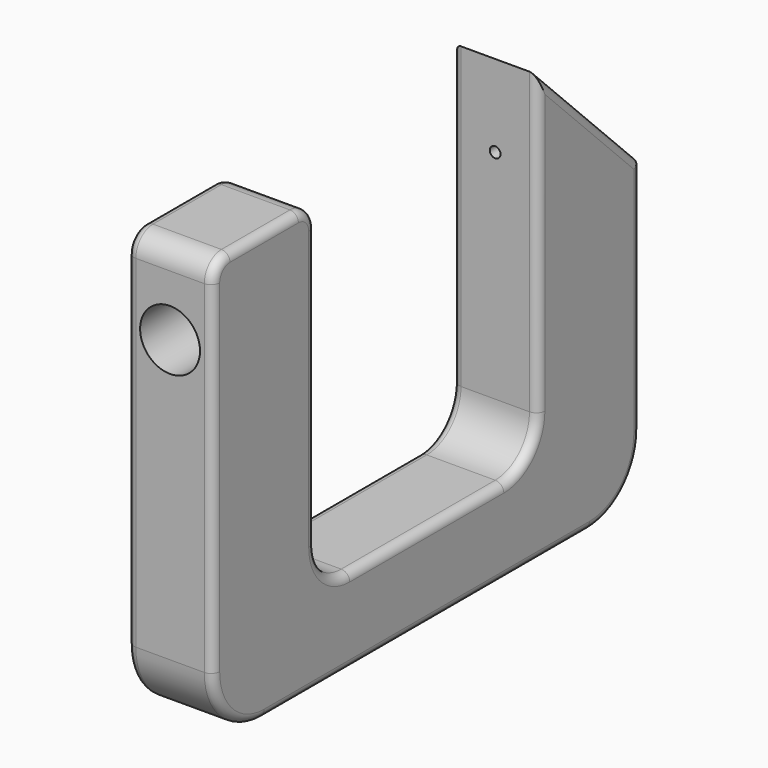
from build123d import *

# Parameters (mm, degrees)
F0_W         = 30
F0_H         = 20
F0_W_2       = 65
F0_H_2       = 80
F1_DEPTH     = 20
F2_R         = 10
F3_SIZE      = 29.99999
F4_T1_DEPTH  = 75
F4_T3_DEPTH  = 52.4263927291
F4_T5_DEPTH  = 80.00001
F4_T7_DEPTH  = 135
F4_T9_DEPTH  = 110
F4_T11_DEPTH = 40
F4_T13_DEPTH = 45
F4_T16_ANGLE = 90
F4_T18_ANGLE = 90
F5_T1_DEPTH  = 40
F5_T3_DEPTH  = 110
F5_T5_DEPTH  = 75
F5_T7_DEPTH  = 45
F5_T9_DEPTH  = 10.00001
F5_T11_DEPTH = 52.4263927291
F5_T13_DEPTH = 80.00001
F5_T15_DEPTH = 135
F5_T18_ANGLE = 90
F5_T20_ANGLE = 90
F6_T1_DEPTH  = 19.9999999998
F6_T4_ANGLE  = 90
F6_T6_ANGLE  = 90
F7_T1_DEPTH  = 19.9999999998
F7_T4_ANGLE  = 90
F7_T6_ANGLE  = 90
F7_T8_ANGLE  = 90
F7_T10_ANGLE = 90
F8_R         = 7
F9_DEPTH     = 52.5
F10_T1_DEPTH = 19.9999999998
F10_T4_ANGLE = 90
F10_T6_ANGLE = 90
F11_R        = 1.25
F12_DEPTH    = 53


# Not quite as in the source:
# - a fillet or chamfer that OpenCascade refuses, or shapes differently, is made with other operations: its cross-section is extruded or revolved along the edge and cut away or added
# - a fillet or chamfer is up to 0.001 mm smaller than in the source, because OpenCascade refuses the exact size


with BuildPart() as f1:
    # F0 (on Right) → F1 (new body)
    with BuildSketch(Plane.YZ):
        with Locations((15, -90)):
            Rectangle(F0_W, F0_H)
        with Locations((62.5, -90)):
            Rectangle(F0_W_2, F0_H)
        with Locations((15, -40)):
            Rectangle(F0_W, F0_H_2)
        with Locations((110, -90)):
            Rectangle(F0_W, F0_H)
        with Locations((110, -40)):
            Rectangle(F0_W, F0_H_2)
    extrude(amount=F1_DEPTH)

    # F2
    f2_edges = [f1.edges().sort_by_distance(p)[0] for p in [
        (10, 95, -80),
        (10, 30, -80),
    ]]
    fillet(f2_edges, radius=F2_R)

    # F3 (size 30 in the source; OpenCascade refuses exactly that, so slightly less here)
    f3_edges = [f1.edges().sort_by_distance(p)[0] for p in [
        (10, 125, 0),
    ]]
    chamfer(f3_edges, length=F3_SIZE)

    # F4: fillet of radius 2 on 10 edges, made by hand

    # F4_s2 → F4_t1 (cut)
    with BuildSketch(Plane.XY.offset(-70)):
        with BuildLine():
            ThreePointArc((18, 95), (19.4142135624, 95.5857864376), (20, 97))
            Line((20, 97), (20, 95))
            Line((20, 95), (18, 95))
        make_face()
        with BuildLine():
            ThreePointArc((18, 30), (19.4142135624, 29.4142135624), (20, 28))
            Line((20, 28), (20, 30))
            Line((20, 30), (18, 30))
        make_face()
    extrude(amount=F4_T1_DEPTH, mode=Mode.SUBTRACT)

    # F4_s4 → F4_t3 (cut)
    with BuildSketch(Plane(origin=(0, 43.9644710941, -43.9644710941), x_dir=(1, 0, 0), z_dir=(0, 0.7071067812, -0.7071067812))):
        with BuildLine():
            ThreePointArc((18, -67.1751512838), (19.4142135624, -66.5893648462), (20, -65.1751512838))
            Line((20, -65.1751512838), (20, -67.1751512838))
            Line((20, -67.1751512838), (18, -67.1751512838))
        make_face()
    extrude(amount=F4_T3_DEPTH, mode=Mode.SUBTRACT)

    # F4_s6 → F4_t5 (cut)
    with BuildSketch(Plane.XY.offset(-105)):
        with BuildLine():
            ThreePointArc((18, 125), (19.4142135624, 124.4142135624), (20, 123))
            Line((20, 123), (20, 125))
            Line((20, 125), (18, 125))
        make_face()
    extrude(amount=F4_T5_DEPTH, mode=Mode.SUBTRACT)

    # F4_s8 → F4_t7 (cut)
    with BuildSketch(Plane.XZ.offset(-130)):
        with BuildLine():
            ThreePointArc((18, -100), (19.4142135624, -99.4142135624), (20, -98))
            Line((20, -98), (20, -100))
            Line((20, -100), (18, -100))
        make_face()
    extrude(amount=F4_T7_DEPTH, mode=Mode.SUBTRACT)

    # F4_s10 → F4_t9 (cut)
    with BuildSketch(Plane.XY.offset(-105)):
        with BuildLine():
            ThreePointArc((18, 0), (19.4142135624, 0.5857864376), (20, 2))
            Line((20, 2), (20, 0))
            Line((20, 0), (18, 0))
        make_face()
    extrude(amount=F4_T9_DEPTH, mode=Mode.SUBTRACT)

    # F4_s12 → F4_t11 (cut)
    with BuildSketch(Plane.XZ.offset(-35)):
        with BuildLine():
            ThreePointArc((18, 0), (19.4142135624, -0.5857864376), (20, -2))
            Line((20, -2), (20, 0))
            Line((20, 0), (18, 0))
        make_face()
    extrude(amount=F4_T11_DEPTH, mode=Mode.SUBTRACT)

    # F4_s14 → F4_t13 (cut)
    with BuildSketch(Plane.XZ.offset(-85)):
        with BuildLine():
            ThreePointArc((18, -80), (19.4142135624, -80.5857864376), (20, -82))
            Line((20, -82), (20, -80))
            Line((20, -80), (18, -80))
        make_face()
    extrude(amount=F4_T13_DEPTH, mode=Mode.SUBTRACT)

    # F4_s15 → F4_t16 (revolve, cut)
    with BuildSketch(Plane.XY.offset(-70)):
        with BuildLine():
            ThreePointArc((18, 95), (19.4142135624, 95.5857864376), (20, 97))
            Line((20, 97), (20, 95))
            Line((20, 95), (18, 95))
        make_face()
    revolve(axis=Axis((20, 85, -70), (-1, 0, 0)), revolution_arc=F4_T16_ANGLE, mode=Mode.SUBTRACT)

    # F4_s17 → F4_t18 (revolve, cut)
    with BuildSketch(Plane.XZ.offset(-40)):
        with BuildLine():
            ThreePointArc((18, -80), (19.4142135624, -80.5857864376), (20, -82))
            Line((20, -82), (20, -80))
            Line((20, -80), (18, -80))
        make_face()
    revolve(axis=Axis((20, 40, -70), (-1, 0, 0)), revolution_arc=F4_T18_ANGLE, mode=Mode.SUBTRACT)

    # F5: fillet of radius 2 on 11 edges, made by hand

    # F5_s2 → F5_t1 (cut)
    with BuildSketch(Plane.XZ.offset(-35)):
        with BuildLine():
            ThreePointArc((0, -2), (0.5857864376, -0.5857864376), (2, 0))
            Line((2, 0), (0, 0))
            Line((0, 0), (0, -2))
        make_face()
    extrude(amount=F5_T1_DEPTH, mode=Mode.SUBTRACT)

    # F5_s4 → F5_t3 (cut)
    with BuildSketch(Plane.XY.offset(-105)):
        with BuildLine():
            ThreePointArc((0, 2), (0.5857864376, 0.5857864376), (2, 0))
            Line((2, 0), (0, 0))
            Line((0, 0), (0, 2))
        make_face()
    extrude(amount=F5_T3_DEPTH, mode=Mode.SUBTRACT)

    # F5_s6 → F5_t5 (cut)
    with BuildSketch(Plane.XY.offset(-70)):
        with BuildLine():
            ThreePointArc((0, 28), (0.5857864376, 29.4142135624), (2, 30))
            Line((2, 30), (0, 30))
            Line((0, 30), (0, 28))
        make_face()
        with BuildLine():
            ThreePointArc((0, 97), (0.5857864376, 95.5857864376), (2, 95))
            Line((2, 95), (0, 95))
            Line((0, 95), (0, 97))
        make_face()
    extrude(amount=F5_T5_DEPTH, mode=Mode.SUBTRACT)

    # F5_s8 → F5_t7 (cut)
    with BuildSketch(Plane.XZ.offset(-85)):
        with BuildLine():
            ThreePointArc((0, -82), (0.5857864376, -80.5857864376), (2, -80))
            Line((2, -80), (0, -80))
            Line((0, -80), (0, -82))
        make_face()
    extrude(amount=F5_T7_DEPTH, mode=Mode.SUBTRACT)

    # F5_s10 → F5_t9 (cut)
    with BuildSketch(Plane.XZ.offset(-100.00001)):
        with BuildLine():
            ThreePointArc((0, -2), (0.5857864376, -0.5857864376), (2, 0))
            Line((2, 0), (0, 0))
            Line((0, 0), (0, -2))
        make_face()
    extrude(amount=F5_T9_DEPTH, mode=Mode.SUBTRACT)

    # F5_s12 → F5_t11 (cut)
    with BuildSketch(Plane(origin=(0, 43.9644710941, -43.9644710941), x_dir=(1, 0, 0), z_dir=(0, 0.7071067812, -0.7071067812))):
        with BuildLine():
            ThreePointArc((0, -65.1751512838), (0.5857864376, -66.5893648462), (2, -67.1751512838))
            Line((2, -67.1751512838), (0, -67.1751512838))
            Line((0, -67.1751512838), (0, -65.1751512838))
        make_face()
    extrude(amount=F5_T11_DEPTH, mode=Mode.SUBTRACT)

    # F5_s14 → F5_t13 (cut)
    with BuildSketch(Plane.XY.offset(-105)):
        with BuildLine():
            ThreePointArc((0, 123), (0.5857864376, 124.4142135624), (2, 125))
            Line((2, 125), (0, 125))
            Line((0, 125), (0, 123))
        make_face()
    extrude(amount=F5_T13_DEPTH, mode=Mode.SUBTRACT)

    # F5_s16 → F5_t15 (cut)
    with BuildSketch(Plane.XZ.offset(-130)):
        with BuildLine():
            ThreePointArc((0, -98), (0.5857864376, -99.4142135624), (2, -100))
            Line((2, -100), (0, -100))
            Line((0, -100), (0, -98))
        make_face()
    extrude(amount=F5_T15_DEPTH, mode=Mode.SUBTRACT)

    # F5_s17 → F5_t18 (revolve, cut)
    with BuildSketch(Plane.XZ.offset(-40)):
        with BuildLine():
            ThreePointArc((0, -82), (0.5857864376, -80.5857864376), (2, -80))
            Line((2, -80), (0, -80))
            Line((0, -80), (0, -82))
        make_face()
    revolve(axis=Axis((0, 40, -70), (-1, 0, 0)), revolution_arc=F5_T18_ANGLE, mode=Mode.SUBTRACT)

    # F5_s19 → F5_t20 (revolve, cut)
    with BuildSketch(Plane.XY.offset(-70)):
        with BuildLine():
            ThreePointArc((0, 97), (0.5857864376, 95.5857864376), (2, 95))
            Line((2, 95), (0, 95))
            Line((0, 95), (0, 97))
        make_face()
    revolve(axis=Axis((0, 85, -70), (-1, 0, 0)), revolution_arc=F5_T20_ANGLE, mode=Mode.SUBTRACT)

    # F6: fillet of radius 5 on 1 edges, made by hand

    # F6_s2 → F6_t1 (cut)
    with BuildSketch(Plane.YZ):
        with BuildLine():
            ThreePointArc((0, -5), (1.4644660941, -1.4644660941), (5, 0))
            Line((5, 0), (0, 0))
            Line((0, 0), (0, -5))
        make_face()
    extrude(amount=F6_T1_DEPTH, mode=Mode.SUBTRACT)

    # F6_s3 → F6_t4 (revolve, cut)
    with BuildSketch(Plane.XY.offset(-5)):
        with BuildLine():
            ThreePointArc((0, 1.9999999999), (0.5857864376, 0.5857864376), (1.9999999999, 0))
            Line((1.9999999999, 0), (0, 0))
            Line((0, 0), (0, 1.9999999999))
        make_face()
    revolve(axis=Axis((0, 5, -5), (-1, 0, 0)), revolution_arc=F6_T4_ANGLE, mode=Mode.SUBTRACT)

    # F6_s5 → F6_t6 (revolve, cut)
    with BuildSketch(Plane.XZ.offset(-5)):
        with BuildLine():
            ThreePointArc((20, -1.9999999999), (19.4142135624, -0.5857864376), (18.0000000001, 0))
            Line((18.0000000001, 0), (20, 0))
            Line((20, 0), (20, -1.9999999999))
        make_face()
    revolve(axis=Axis((20, 5, -5), (1, 0, 0)), revolution_arc=F6_T6_ANGLE, mode=Mode.SUBTRACT)

    # F7: fillet of radius 15 on 2 edges, made by hand

    # F7_s2 → F7_t1 (cut)
    with BuildSketch(Plane.YZ):
        with BuildLine():
            ThreePointArc((15, -100), (4.3933982822, -95.6066017178), (0, -85))
            Line((0, -85), (0, -100))
            Line((0, -100), (15, -100))
        make_face()
        with BuildLine():
            ThreePointArc((125, -85), (120.6066017178, -95.6066017178), (110, -100))
            Line((110, -100), (125, -100))
            Line((125, -100), (125, -85))
        make_face()
    extrude(amount=F7_T1_DEPTH, mode=Mode.SUBTRACT)

    # F7_s3 → F7_t4 (revolve, cut)
    with BuildSketch(Plane.XY.offset(-85)):
        with BuildLine():
            ThreePointArc((0, 123.0000000001), (0.5857864376, 124.4142135624), (1.9999999999, 125))
            Line((1.9999999999, 125), (0, 125))
            Line((0, 125), (0, 123.0000000001))
        make_face()
    revolve(axis=Axis((0, 110, -85), (-1, 0, 0)), revolution_arc=F7_T4_ANGLE, mode=Mode.SUBTRACT)

    # F7_s5 → F7_t6 (revolve, cut)
    with BuildSketch(Plane.XZ.offset(-110)):
        with BuildLine():
            ThreePointArc((20, -98.0000000001), (19.4142135624, -99.4142135624), (18.0000000001, -100))
            Line((18.0000000001, -100), (20, -100))
            Line((20, -100), (20, -98.0000000001))
        make_face()
    revolve(axis=Axis((20, 110, -85), (1, 0, 0)), revolution_arc=F7_T6_ANGLE, mode=Mode.SUBTRACT)

    # F7_s7 → F7_t8 (revolve, cut)
    with BuildSketch(Plane.XZ.offset(-15)):
        with BuildLine():
            ThreePointArc((0, -98.0000000001), (0.5857864376, -99.4142135624), (1.9999999999, -100))
            Line((1.9999999999, -100), (0, -100))
            Line((0, -100), (0, -98.0000000001))
        make_face()
    revolve(axis=Axis((0, 15, -85), (-1, 0, 0)), revolution_arc=F7_T8_ANGLE, mode=Mode.SUBTRACT)

    # F7_s9 → F7_t10 (revolve, cut)
    with BuildSketch(Plane.XY.offset(-85)):
        with BuildLine():
            ThreePointArc((20, 1.9999999999), (19.4142135624, 0.5857864376), (18.0000000001, 0))
            Line((18.0000000001, 0), (20, 0))
            Line((20, 0), (20, 1.9999999999))
        make_face()
    revolve(axis=Axis((20, 15, -85), (1, 0, 0)), revolution_arc=F7_T10_ANGLE, mode=Mode.SUBTRACT)

    # F8 (on face) → F9 (cut)
    with BuildSketch(Plane.XZ):
        with Locations((10, -19.1889982671)):
            Circle(F8_R)
    extrude(amount=-F9_DEPTH, mode=Mode.SUBTRACT)

    # F10: fillet of radius 5 on 1 edges, made by hand

    # F10_s2 → F10_t1 (cut)
    with BuildSketch(Plane.YZ):
        with BuildLine():
            ThreePointArc((25, 0), (28.5355339059, -1.4644660941), (30, -5))
            Line((30, -5), (30, 0))
            Line((30, 0), (25, 0))
        make_face()
    extrude(amount=F10_T1_DEPTH, mode=Mode.SUBTRACT)

    # F10_s3 → F10_t4 (revolve, cut)
    with BuildSketch(Plane.XZ.offset(-25)):
        with BuildLine():
            ThreePointArc((0, -1.9999999999), (0.5857864376, -0.5857864376), (1.9999999999, 0))
            Line((1.9999999999, 0), (0, 0))
            Line((0, 0), (0, -1.9999999999))
        make_face()
    revolve(axis=Axis((0, 25, -5), (-1, 0, 0)), revolution_arc=F10_T4_ANGLE, mode=Mode.SUBTRACT)

    # F10_s5 → F10_t6 (revolve, cut)
    with BuildSketch(Plane.XY.offset(-5)):
        with BuildLine():
            ThreePointArc((20, 28.0000000001), (19.4142135624, 29.4142135624), (18.0000000001, 30))
            Line((18.0000000001, 30), (20, 30))
            Line((20, 30), (20, 28.0000000001))
        make_face()
    revolve(axis=Axis((20, 25, -5), (1, 0, 0)), revolution_arc=F10_T6_ANGLE, mode=Mode.SUBTRACT)

    # F11 (on face) → F12 (cut)
    with BuildSketch(Plane.XZ.offset(-95)):
        with Locations((9.9868811667, -19.1981494427)):
            Circle(F11_R)
    extrude(amount=-F12_DEPTH, mode=Mode.SUBTRACT)


solid = f1.part
